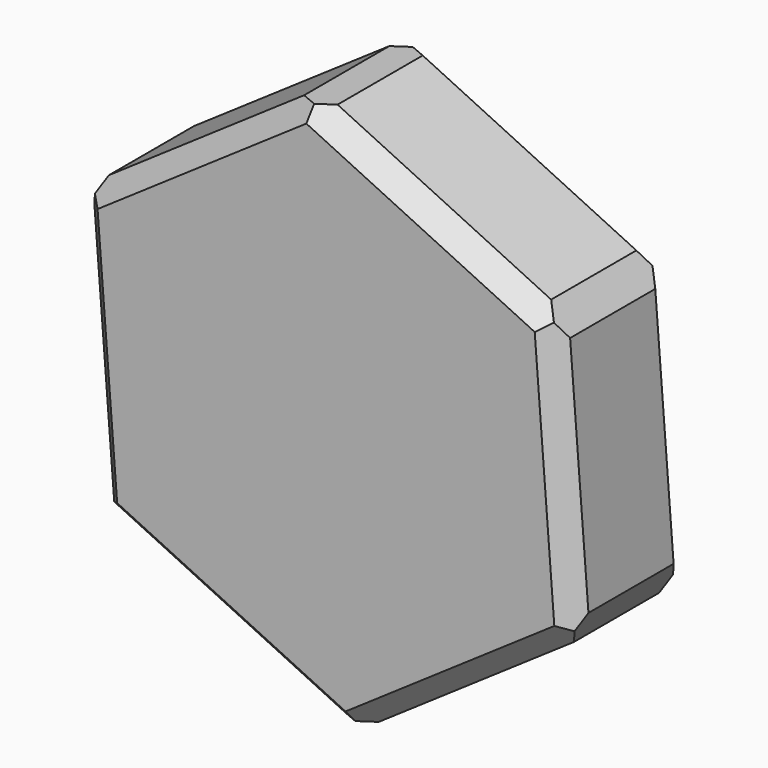
from build123d import *

# Parameters (mm, degrees)
F1_DEPTH = 38.1
F2_SIZE  = 5.08
F3_SIZE  = 5.08
F4_SIZE  = 5.08
F5_SIZE  = 5.08
F6_SIZE  = 5.08


# Not quite as in the source:
# - the program builds the solid bodies; features that only make, move or delete a surface that nothing else refers to are left out


with BuildPart() as f1:
    # F0 (on Front) → F1 (new body)
    with BuildSketch(Plane.XZ):
        Polygon((5.5975063319, -72.0986601401), (65.238024426, -31.2017473888), (59.6405180942, 40.8969127513), (-5.5975063319, 72.0986601401), (-65.238024426, 31.2017473888), (-59.6405180942, -40.8969127513), align=None)
    extrude(amount=F1_DEPTH)

    # F2
    f2_edges = [f1.edges().sort_by_distance(p)[0] for p in [
        (27.021506, -38.1, 56.497786),
    ]]
    chamfer(f2_edges, length=F2_SIZE)

    # F3
    f3_edges = [f1.edges().sort_by_distance(p)[0] for p in [
        (62.666292, -38.1, 1.923443),
    ]]
    chamfer(f3_edges, length=F3_SIZE)

    # F4
    f4_edges = [f1.edges().sort_by_distance(p)[0] for p in [
        (-62.439271, 0, -4.847583),
        (62.439271, 0, 4.847583),
        (-27.021506, 0, -56.497786),
        (32.998896, -38.1, -53.30888),
        (-35.417765, 0, 51.650204),
        (-27.021506, -38.1, -56.497786),
        (27.021506, 0, 56.497786),
        (-62.439271, -38.1, -4.847583),
        (35.417765, 0, -51.650204),
        (-37.836635, -38.1, 49.991528),
    ]]
    chamfer(f4_edges, length=F4_SIZE)

    # F5
    f5_edges = [f1.edges().sort_by_distance(p)[0] for p in [
        (5.597506, -19.05, -72.09866),
    ]]
    chamfer(f5_edges, length=F5_SIZE)

    # F6
    f6_edges = [f1.edges().sort_by_distance(p)[0] for p in [
        (-5.597506, -19.05, 72.09866),
        (-65.238024, -19.05, 31.201747),
        (65.238024, -19.05, -31.201747),
        (59.640518, -19.05, 40.896913),
    ]]
    chamfer(f6_edges, length=F6_SIZE)


solid = f1.part
